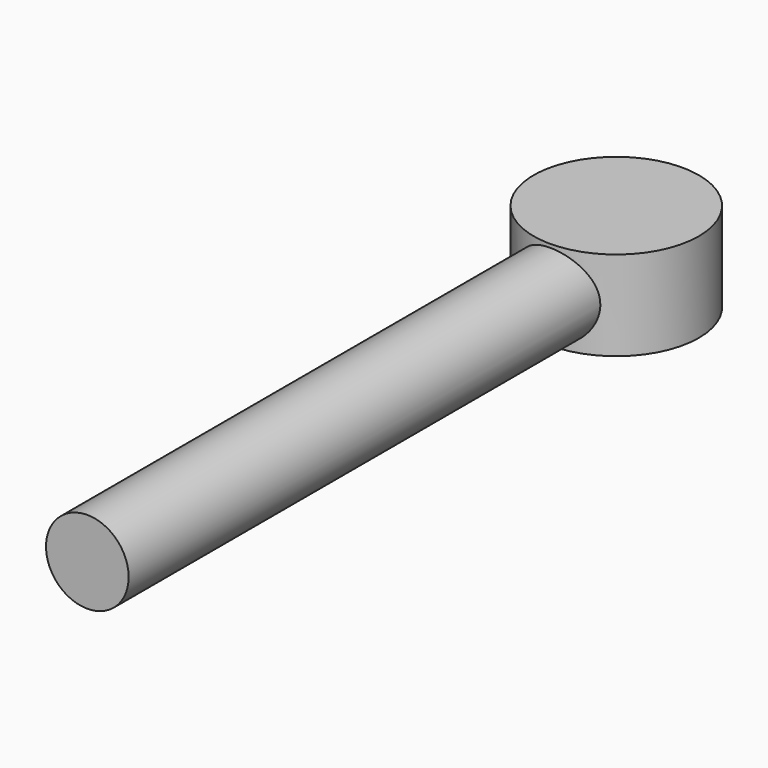
from build123d import *

# Parameters (mm, degrees)
F0_R     = 19.05
F1_DEPTH = 20.6375
F2_R     = 9.525
F3_DEPTH = 152.4


# Not quite as in the source:
# - a length typed as a fraction of an inch, garbled in the dataset ("3 / 203.2 mm" for 3/8 in), is restored


with BuildPart() as f1:
    # F0 (on Top) → F1 (new body)
    with BuildSketch(Plane.XY):
        Circle(F0_R)
    extrude(amount=F1_DEPTH)

    # F2 (on Front) → F3 (join)
    with BuildSketch(Plane.XZ):
        with Locations((0, 10.31875)):
            Circle(F2_R)
    extrude(amount=F3_DEPTH)


solid = f1.part
